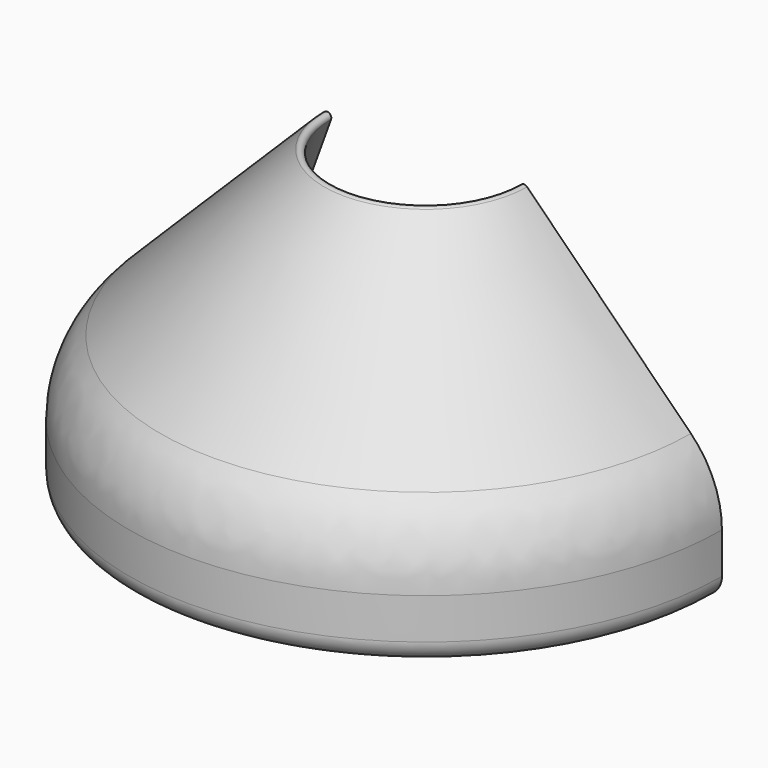
from build123d import *

# Parameters (mm, degrees)
F1_ANGLE    = 180
F2_R        = 5
F3_R        = 1
F4_T2_ANGLE = 242.2675380927


# Not quite as in the source:
# - a fillet or chamfer that OpenCascade refuses, or shapes differently, is made with other operations: its cross-section is extruded or revolved along the edge and cut away or added


with BuildPart() as f1:
    # F0 (on Front) → F1 (revolve)
    with BuildSketch(Plane.XZ):
        Polygon((14, -25), (4.157225346, -15.157225346), (7.7397023427, -25), (7.7397023427, -30), (14, -30), align=None)
    revolve(axis=Axis((0, 0, 0), (0, 0, -1)), revolution_arc=F1_ANGLE)

    # F2
    f2_edges = [f1.edges().sort_by_distance(p)[0] for p in [
        (0, -14, -25),
    ]]
    fillet(f2_edges, radius=F2_R)

    # F3
    f3_edges = [f1.edges().sort_by_distance(p)[0] for p in [
        (0, -14, -30),
        (0, -7.739702, -30),
    ]]
    fillet(f3_edges, radius=F3_R)

    # F4: fillet of radius 0.2 on 1 edges, made by hand

    # F4_s1 → F4_t2 (revolve, cut)
    with BuildSketch(Plane(origin=(0, 0, 0), x_dir=(0, 0, 1), z_dir=(-0.5170379067, 0.8559625009, 0))):
        with BuildLine():
            ThreePointArc((-15.7951358602, 4.7951358602), (-15.7678789273, 4.5462545823), (-16.0049612451, 4.4657759798))
            Line((-16.0049612451, 4.4657759798), (-15.157225346, 4.157225346))
            Line((-15.157225346, 4.157225346), (-15.7951358602, 4.7951358602))
        make_face()
    revolve(axis=Axis((0, 0, -15.157225346), (0, 0, -1)), revolution_arc=F4_T2_ANGLE, mode=Mode.SUBTRACT)


solid = f1.part
